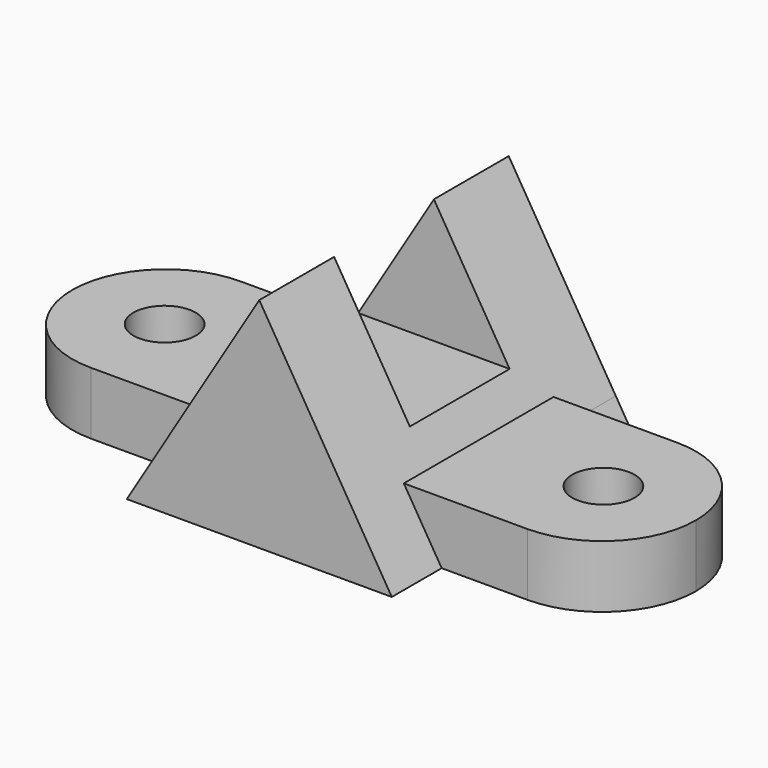
from build123d import *

# Parameters (mm, degrees)
F0_W      = 127
F0_H      = 38.1
F1_DEPTH  = 12.7
F3_DEPTH  = 50.8
F5_DEPTH  = 12.7
F6_R      = 19.04999
F8_D      = 12.7
F11_D     = 12.7
F12_W     = 25.4
F12_H     = 25.4
F13_DEPTH = 25.4


# Not quite as in the source:
# - a fillet or chamfer is up to 0.001 mm smaller than in the source, because OpenCascade refuses the exact size


with BuildPart() as f1:
    # F0 (on Top) → F1 (new body)
    with BuildSketch(Plane.XY):
        with Locations((63.5, 19.05)):
            Rectangle(F0_W, F0_H)
    extrude(amount=F1_DEPTH)

    # F2 (on face) → F3 (join)
    with BuildSketch(Plane.XZ):
        Polygon((63.5, 12.7), (63.5, 6.35), (85.3080808081, 8.5308080808), (82.7767857143, 12.7), align=None)
        Polygon((85.3080808081, 8.5308080808), (63.5, 6.35), (88.1273764259, 3.8872623574), align=None)
        Polygon((63.5, 6.35), (63.5, 0), (90.4875, 0), (88.1273764259, 3.8872623574), align=None)
        Polygon((38.8726235741, 3.8872623574), (36.5125, 0), (63.5, 0), (63.5, 6.35), align=None)
        Polygon((41.6919191919, 8.5308080808), (38.8726235741, 3.8872623574), (63.5, 6.35), align=None)
        Polygon((63.5, 12.7), (44.2232142857, 12.7), (41.6919191919, 8.5308080808), (63.5, 6.35), align=None)
        Polygon((63.5, 44.45), (44.2232142857, 12.7), (63.5, 12.7), align=None)
        Polygon((63.5, 44.45), (63.5, 12.7), (82.7767857143, 12.7), align=None)
    extrude(amount=-F3_DEPTH)

    # F4 (on face) → F5 (join)
    with BuildSketch(Plane.XZ):
        Polygon((90.4875, 0), (63.5, 44.45), (36.5125, 0), align=None)
    extrude(amount=F5_DEPTH)

    # F6 (radius 19.05 in the source; OpenCascade refuses exactly that, so slightly less here)
    f6_edges = [f1.edges().sort_by_distance(p)[0] for p in [
        (0, 0, 6.35),
        (0, 38.1, 6.35),
        (127, 38.1, 6.35),
        (127, 0, 6.35),
    ]]
    fillet(f6_edges, radius=F6_R)

    # F8 (through all)
    with Locations(Plane.XY.offset(12.7)):
        with Locations((18.8232142857, 19.05)):
            Hole(F8_D / 2)

    # F11 (through all)
    with Locations(Plane.XY.offset(12.7)):
        with Locations((108.1767857143, 19.05)):
            Hole(F11_D / 2)

    # F12 (on offset) → F13 (cut, symmetric)
    with BuildSketch(Plane.YZ.offset(63.5)):
        with Locations((19.05, 31.75)):
            Rectangle(F12_W, F12_H)
    extrude(amount=F13_DEPTH, both=True, mode=Mode.SUBTRACT)


solid = f1.part
